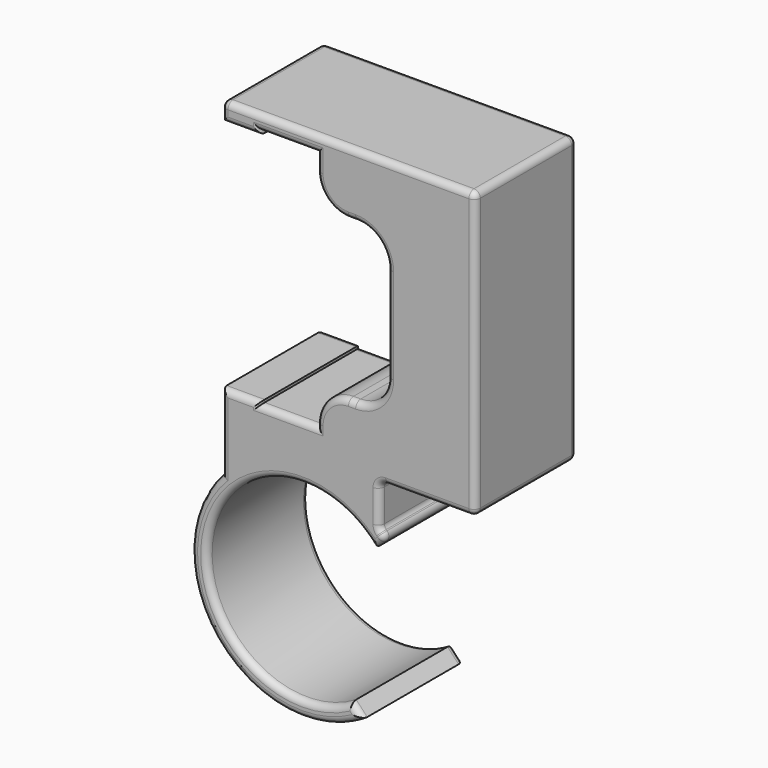
from build123d import *

# Parameters (mm, degrees)
F1_DEPTH = 20
F3_DEPTH = 20
F4_R     = 5
F5_R     = 1


# Not quite as in the source:
# - a feature names something its author has since deleted; it is built from what else it names


with BuildPart() as f1:
    # F0 (on Front) → F1 (new body)
    with BuildSketch(Plane.XZ):
        with BuildLine():
            ThreePointArc((7.7246587161, -12.8580576962), (-14.8017953762, 2.4304019506), (11.4307152083, 9.7128136926))
            Line((11.4307152083, 9.7128136926), (13.2814653766, 11.3952918984))
            ThreePointArc((13.2814653766, 11.3952918984), (12.7404924616, 11.9970768038), (12.1722789481, 12.5732106166))
            Line((12.1722789481, 12.5732106166), (12.1722789481, 17.5))
            Line((12.1722789481, 17.5), (12.1722789481, 19.1013980657))
            Line((12.1722789481, 19.1013980657), (-12.6995956525, 19.1013980657))
            Line((-12.6995956525, 19.1013980657), (-12.6995956525, 17.5))
            Line((-12.6995956525, 17.5), (-12.6995956525, 12.0403600554))
            ThreePointArc((-12.6995956525, 12.0403600554), (-13.4761736825, -11.1643514311), (9.4680293839, -14.71755481))
            Line((9.4680293839, -14.71755481), (7.7246587161, -12.8580576962))
        make_face()
    extrude(amount=F1_DEPTH)

    # F2 (on face) → F3 (join)
    with BuildSketch(Plane(origin=(0, 0, 0), x_dir=(-1, 0, 0), z_dir=(0, 1, 0))):
        Polygon((-12.1722789481, 19.1013980657), (12.6995956525, 19.1013980657), (12.6995956525, 24.1013980657), (6.6995956525, 24.1013980657), (6.6995956525, 23.6930285978), (-2.3004043475, 23.6930285978), (-2.3004043475, 29.1013980657), (-13.4298764169, 29.1013980657), (-13.4298764169, 54.1013980657), (-2.3004043475, 54.1013980657), (-2.3004043475, 61.6930285978), (6.6995956525, 61.6930285978), (6.6995956525, 61.1013980657), (12.6995956525, 61.1013980657), (12.6995956525, 64.1013980657), (-27.3004043475, 64.1013980657), (-27.3004043475, 19.1013980657), align=None)
    extrude(amount=-F3_DEPTH)

    # F4
    f4_edges = [f1.edges().sort_by_distance(p)[0] for p in [
        (2.300404, -10, 54.101398),
        (2.300404, -10, 29.101398),
        (13.429876, -10, 54.101398),
        (13.429876, -10, 29.101398),
    ]]
    fillet(f4_edges, radius=F4_R)

    # F5
    f5_edges = [f1.edges().sort_by_distance(p)[0] for p in [
        (2.300404, 0, 60.397213),
        (3.76487, 0, 55.565864),
        (-2.199596, 0, 61.693029),
        (7.86514, 0, 54.101398),
        (-6.699596, 0, 61.397213),
        (11.96541, 0, 52.636932),
        (-9.699596, 0, 61.101398),
        (13.429876, 0, 41.601398),
        (-12.699596, 0, 62.601398),
        (11.96541, 0, 30.565864),
        (7.300404, 0, 64.101398),
        (7.86514, 0, 29.101398),
        (27.300404, 0, 41.601398),
        (3.76487, 0, 27.636932),
        (19.736342, 0, 19.101398),
        (2.300404, 0, 23.897213),
        (12.172279, 0, 15.837304),
        (-2.199596, 0, 23.693029),
        (12.740492, 0, 11.997077),
        (-6.699596, 0, 23.897213),
        (12.35609, 0, 10.554053),
        (-9.699596, 0, 24.101398),
        (-14.801795, 0, 2.430402),
        (-12.699596, 0, 18.070879),
        (8.596344, 0, -13.787806),
        (-13.476174, 0, -11.164351),
        (2.300404, -20, 60.397213),
        (3.76487, -20, 55.565864),
        (-2.199596, -20, 61.693029),
        (7.86514, -20, 54.101398),
        (-6.699596, -20, 61.397213),
        (11.96541, -20, 52.636932),
        (-9.699596, -20, 61.101398),
        (13.429876, -20, 41.601398),
        (-12.699596, -20, 62.601398),
        (11.96541, -20, 30.565864),
        (7.300404, -20, 64.101398),
        (7.86514, -20, 29.101398),
        (27.300404, -20, 41.601398),
        (3.76487, -20, 27.636932),
        (19.736342, -20, 19.101398),
        (2.300404, -20, 23.897213),
        (12.172279, -20, 15.837304),
        (-2.199596, -20, 23.693029),
        (12.740492, -20, 11.997077),
        (-6.699596, -20, 23.897213),
        (12.35609, -20, 10.554053),
        (-9.699596, -20, 24.101398),
        (-14.801795, -20, 2.430402),
        (-12.699596, -20, 18.070879),
        (8.596344, -20, -13.787806),
        (-13.476174, -20, -11.164351),
        (-12.699596, -10, 64.101398),
        (27.300404, -10, 64.101398),
        (27.300404, -10, 19.101398),
        (12.172279, -10, 19.101398),
        (12.172279, -10, 12.573211),
        (13.281465, -10, 11.395292),
    ]]
    fillet(f5_edges, radius=F5_R)


solid = f1.part
